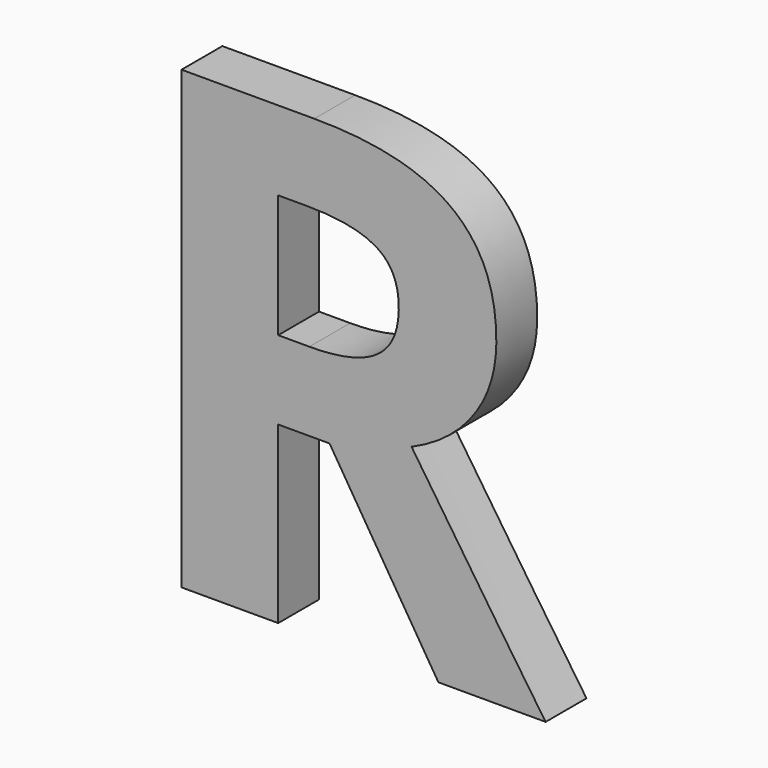
from build123d import *

# Parameters (mm, degrees)
F0_TEXT_SIZE = 62.5
F1_DEPTH     = 5


# Not quite as in the source:
# - Text() gives the source's letters only with a copy of the font that has no kerning and outlines rounded to 1/6400 em; it was checked with that copy


with BuildPart() as f1:
    # F0 (on Front) → F1 (new body)
    with BuildSketch(Plane.XZ):
        with Locations((-60.0394800157, 12.0789487609)):
            Text('R', F0_TEXT_SIZE, font='Open Sans', font_style=FontStyle.BOLD, text_align=(TextAlign.LEFT, TextAlign.BOTTOM))
    extrude(amount=F1_DEPTH)


solid = f1.part
